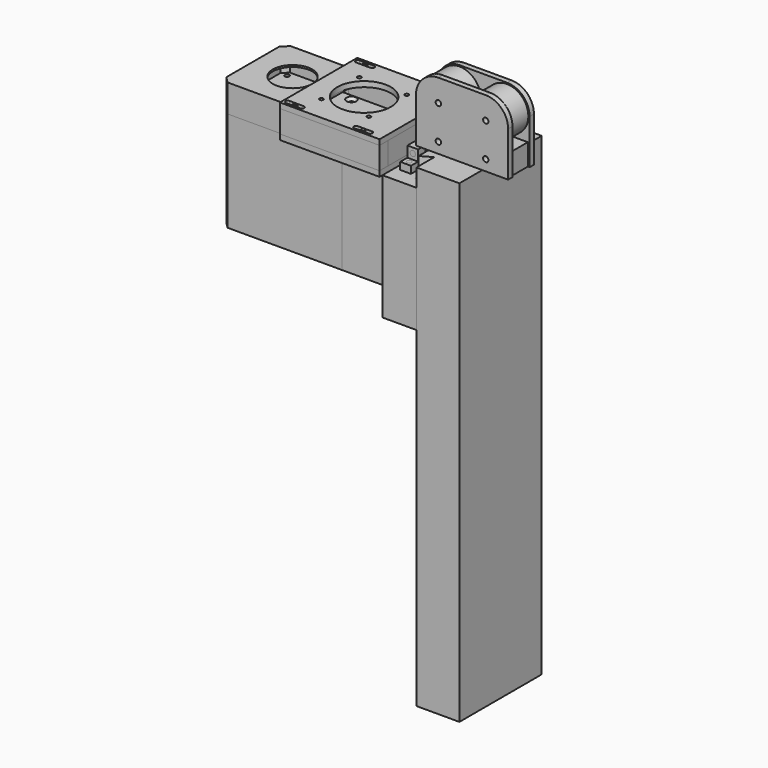
from build123d import *

# Parameters (mm, degrees)
F4_DEPTH       = 140
F1_W           = 50
F1_H           = 88
F1_R           = 2.5
F1_W_2         = 12
F1_H_2         = 10
F5_DEPTH       = 112
F1_R_2         = 25
F1_R_3         = 20
F6_DEPTH       = 112
F7_DEPTH       = 9.5
F8_DEPTH       = 9.5
F9_DEPTH       = 20
F2_R           = 2.5
F2_R_2         = 2.1
F2_R_3         = 6
F10_DEPTH      = 6
F11_SIZE       = 3
F3_W           = 101.8
F3_H           = 2
F3_W_2         = 9.6
F3_H_2         = 10
F3_R           = 2.1
F12_DEPTH      = 25
F3_H_3         = 84
F3_R_2         = 30
F13_DEPTH      = 6
F14_DEPTH      = 6
F14_DEPTH_BACK = 25
F15_DEPTH      = 25
F16_DEPTH      = 29
F17_R          = 25
F17_R_2        = 22
F18_DEPTH      = 2
F19_DEPTH      = 6
F21_DEPTH      = 1
F22_DEPTH      = 8
F23_DEPTH      = 20
F24_R          = 3
F25_DEPTH      = 45
F26_DEPTH      = 10
F27_DEPTH      = 8
F28_DEPTH      = 45
F30_DEPTH      = 20
F30_DEPTH_BACK = 510
F31_DEPTH      = 140
F29_W          = 5
F29_H          = 12.5
F29_W_2        = 2
F29_H_2        = 7.5
F32_DEPTH      = 380
F34_DEPTH      = 50
F35_R          = 24
F35_W          = 99
F35_H          = 24
F35_R_2        = 3
F35_R_3        = 11
F35_R_4        = 10
F35_R_5        = 4
F35_W_2        = 2
F36_DEPTH      = 18
F37_DEPTH      = 12
F38_DEPTH      = 12
F39_DEPTH      = 11.5
F40_DEPTH      = 5.5


with BuildPart() as f4:
    # F1 (on Top) → F4 (new body)
    with BuildSketch(Plane.XY):
        Polygon((0, -20), (0, 0), (-38, 0), (-38, -6), (-38, -94), (-38, -100), (0, -100), (0, -80), (-12.124355653, -87), (-12.124355653, -60), (-20.124355653, -60), (-20.124355653, -62.5), (-20.124355653, -72.5), (-20.124355653, -82.5), (-32.124355653, -82.5), (-32.124355653, -72.5), (-32.124355653, -62.5), (-32.124355653, -37.5), (-32.124355653, -27.5), (-32.124355653, -17.5), (-20.124355653, -17.5), (-20.124355653, -27.5), (-20.124355653, -35), (-12.124355653, -35), (-12.124355653, -13), align=None)
    extrude(amount=-F4_DEPTH)

    # F1 (on Top) → F5 (join)
    with BuildSketch(Plane.XY):
        with Locations((-63, -50)):
            Rectangle(F1_W, F1_H)
        with Locations((-55.6, -86)):
            Circle(F1_R, mode=Mode.SUBTRACT)
        with Locations((-55.6, -14)):
            Circle(F1_R, mode=Mode.SUBTRACT)
        Polygon((-20.124355653, -60), (-20.124355653, -37.5), (-32.124355653, -37.5), (-32.124355653, -62.5), (-20.124355653, -62.5), align=None)
        with Locations((-26.124355653, -50)):
            Circle(F1_R, mode=Mode.SUBTRACT)
        with Locations((-26.124355653, -77.5)):
            Rectangle(F1_W_2, F1_H_2)
        with Locations((-26.124355653, -77.5)):
            Circle(F1_R, mode=Mode.SUBTRACT)
        with Locations((-26.124355653, -22.5)):
            Rectangle(F1_W_2, F1_H_2)
        with Locations((-26.124355653, -22.5)):
            Circle(F1_R, mode=Mode.SUBTRACT)
        with Locations((-26.124355653, -67.5)):
            Rectangle(F1_W_2, F1_H_2)
        Polygon((-20.124355653, -37.5), (-20.124355653, -35), (-20.124355653, -27.5), (-32.124355653, -27.5), (-32.124355653, -37.5), align=None)
        with Locations((-55.6, -86)):
            Circle(F1_R)
        with Locations((-55.6, -14)):
            Circle(F1_R)
        with Locations((-26.124355653, -77.5)):
            Circle(F1_R)
        with Locations((-26.124355653, -50)):
            Circle(F1_R)
        with Locations((-26.124355653, -22.5)):
            Circle(F1_R)
    extrude(amount=-F5_DEPTH)


with BuildPart() as f6:
    # F1 (on Top) → F6 (new body)
    with BuildSketch(Plane.XY):
        Polygon((-88, -94), (-88, -6), (-215.9289321881, -6), (-223, -13.0710678119), (-223, -86.9289321881), (-215.9289321881, -94), align=None)
        with Locations((-213.4, -86)):
            Circle(F1_R, mode=Mode.SUBTRACT)
        with Locations((-141.4, -86)):
            Circle(F1_R, mode=Mode.SUBTRACT)
        with BuildLine():
            ThreePointArc((-140.061745502, -35.7346366626), (-126.6088552227, -37.8642844766), (-120.425, -50))
            ThreePointArc((-120.425, -50), (-126.6088552227, -62.1357155234), (-140.061745502, -64.2653633374))
            ThreePointArc((-140.061745502, -64.2653633374), (-219.5, -50), (-140.061745502, -35.7346366626))
        make_face(mode=Mode.SUBTRACT)
        with Locations((-213.4, -14)):
            Circle(F1_R, mode=Mode.SUBTRACT)
        with Locations((-141.4, -14)):
            Circle(F1_R, mode=Mode.SUBTRACT)
        with BuildLine():
            ThreePointArc((-140.061745502, -64.2653633374), (-150.425, -50), (-140.061745502, -35.7346366626))
            ThreePointArc((-140.061745502, -35.7346366626), (-219.5, -50), (-140.061745502, -64.2653633374))
        make_face()
        with Locations((-178.5, -50)):
            Circle(F1_R_2, mode=Mode.SUBTRACT)
        with BuildLine():
            ThreePointArc((-137.5, -50), (-138.1455180035, -42.7532225927), (-140.061745502, -35.7346366626))
            ThreePointArc((-140.061745502, -35.7346366626), (-150.425, -50), (-140.061745502, -64.2653633374))
            ThreePointArc((-140.061745502, -64.2653633374), (-138.1455180035, -57.2467774073), (-137.5, -50))
        make_face()
        with Locations((-178.5, -50)):
            Circle(F1_R_2)
        with Locations((-178.5, -50)):
            Circle(F1_R_3, mode=Mode.SUBTRACT)
        with BuildLine():
            ThreePointArc((-140.061745502, -64.2653633374), (-126.6088552227, -62.1357155234), (-120.425, -50))
            ThreePointArc((-120.425, -50), (-126.6088552227, -37.8642844766), (-140.061745502, -35.7346366626))
            ThreePointArc((-140.061745502, -35.7346366626), (-138.1455180035, -42.7532225927), (-137.5, -50))
            ThreePointArc((-137.5, -50), (-138.1455180035, -57.2467774073), (-140.061745502, -64.2653633374))
        make_face()
        with Locations((-141.4, -86)):
            Circle(F1_R)
        with Locations((-141.4, -14)):
            Circle(F1_R)
        with Locations((-213.4, -14)):
            Circle(F1_R)
        with Locations((-213.4, -86)):
            Circle(F1_R)
    extrude(amount=-F6_DEPTH)

    # F1 (on Top) → F7 (cut)
    with BuildSketch(Plane.XY):
        with BuildLine():
            ThreePointArc((-140.061745502, -64.2653633374), (-150.425, -50), (-140.061745502, -35.7346366626))
            ThreePointArc((-140.061745502, -35.7346366626), (-219.5, -50), (-140.061745502, -64.2653633374))
        make_face()
        with Locations((-178.5, -50)):
            Circle(F1_R_2, mode=Mode.SUBTRACT)
        with BuildLine():
            ThreePointArc((-137.5, -50), (-138.1455180035, -42.7532225927), (-140.061745502, -35.7346366626))
            ThreePointArc((-140.061745502, -35.7346366626), (-150.425, -50), (-140.061745502, -64.2653633374))
            ThreePointArc((-140.061745502, -64.2653633374), (-138.1455180035, -57.2467774073), (-137.5, -50))
        make_face()
        with BuildLine():
            ThreePointArc((-140.061745502, -64.2653633374), (-126.6088552227, -62.1357155234), (-120.425, -50))
            ThreePointArc((-120.425, -50), (-126.6088552227, -37.8642844766), (-140.061745502, -35.7346366626))
            ThreePointArc((-140.061745502, -35.7346366626), (-138.1455180035, -42.7532225927), (-137.5, -50))
            ThreePointArc((-137.5, -50), (-138.1455180035, -57.2467774073), (-140.061745502, -64.2653633374))
        make_face()
        with Locations((-178.5, -50)):
            Circle(F1_R_2)
        with Locations((-178.5, -50)):
            Circle(F1_R_3, mode=Mode.SUBTRACT)
    extrude(amount=-F7_DEPTH, mode=Mode.SUBTRACT)


with BuildPart() as f8:
    # F1 (on Top) → F8 (new body, through all)
    with BuildSketch(Plane.XY):
        with BuildLine():
            ThreePointArc((-140.061745502, -64.2653633374), (-150.425, -50), (-140.061745502, -35.7346366626))
            ThreePointArc((-140.061745502, -35.7346366626), (-219.5, -50), (-140.061745502, -64.2653633374))
        make_face()
        with Locations((-178.5, -50)):
            Circle(F1_R_2, mode=Mode.SUBTRACT)
    extrude(amount=-F8_DEPTH)


with BuildPart() as f9_tool:
    # F1 (on Top) → F9 (new body)
    with BuildSketch(Plane.XY):
        with Locations((-213.4, -14)):
            Circle(F1_R)
        with Locations((-55.6, -14)):
            Circle(F1_R)
        with Locations((-55.6, -86)):
            Circle(F1_R)
        with Locations((-213.4, -86)):
            Circle(F1_R)
        with Locations((-141.4, -86)):
            Circle(F1_R)
        with Locations((-141.4, -14)):
            Circle(F1_R)
    extrude(amount=-F9_DEPTH)


with BuildPart() as f4_1:
    add(f4.part)

    # F9: cut by f9_tool
    add(f9_tool.part, mode=Mode.SUBTRACT)

    # F1 (on Top) → F26 (cut)
    with BuildSketch(Plane.XY):
        with Locations((-26.124355653, -77.5)):
            Circle(F1_R)
        with Locations((-26.124355653, -50)):
            Circle(F1_R)
        with Locations((-26.124355653, -22.5)):
            Circle(F1_R)
    extrude(amount=-F26_DEPTH, mode=Mode.SUBTRACT)


with BuildPart() as f6_1:
    add(f6.part)

    # F9: cut by f9_tool
    add(f9_tool.part, mode=Mode.SUBTRACT)


with BuildPart() as f10:
    # F2 (on Top) → F10 (new body)
    with BuildSketch(Plane.XY):
        with BuildLine():
            Line((-175.5, -25), (-175.5, -8))
            Line((-175.5, -8), (-181.5, -8))
            Line((-181.5, -8), (-181.5, -25.180652708))
            ThreePointArc((-181.5, -25.180652708), (-180.0027171558, -25.0452040451), (-178.5, -25))
            Line((-178.5, -25), (-175.5, -25))
        make_face()
        with BuildLine():
            Line((-47.6, -6), (-88, -6))
            Line((-88, -6), (-149.4, -6))
            Line((-149.4, -6), (-149.4, -8))
            Line((-149.4, -8), (-175.5, -8))
            Line((-175.5, -8), (-175.5, -25))
            Line((-175.5, -25), (-98.5, -25))
            ThreePointArc((-98.5, -25), (-80.8223304703, -32.3223304703), (-73.5, -50))
            ThreePointArc((-73.5, -50), (-80.8223304703, -67.6776695297), (-98.5, -75))
            Line((-98.5, -75), (-178.5, -75))
            ThreePointArc((-178.5, -75), (-203.4547959549, -51.5027171558), (-181.5, -25.180652708))
            Line((-181.5, -25.180652708), (-181.5, -8))
            Line((-181.5, -8), (-215.1005050634, -8))
            Line((-215.1005050634, -8), (-221, -13.8994949366))
            Line((-221, -13.8994949366), (-221, -86.1005050634))
            Line((-221, -86.1005050634), (-215.1005050634, -92))
            Line((-215.1005050634, -92), (-149.4, -92))
            Line((-149.4, -92), (-149.4, -94))
            Line((-149.4, -94), (-88, -94))
            Line((-88, -94), (-47.6, -94))
            Line((-47.6, -94), (-47.6, -6))
        make_face()
        with Locations((-213.4, -86)):
            Circle(F2_R, mode=Mode.SUBTRACT)
        with Locations((-141.4, -86)):
            Circle(F2_R, mode=Mode.SUBTRACT)
        with Locations((-55.6, -86)):
            Circle(F2_R, mode=Mode.SUBTRACT)
        with Locations((-213.4, -14)):
            Circle(F2_R, mode=Mode.SUBTRACT)
        with Locations((-141.4, -14)):
            Circle(F2_R, mode=Mode.SUBTRACT)
        with Locations((-55.6, -14)):
            Circle(F2_R, mode=Mode.SUBTRACT)
        Polygon((-149.4, -6), (-88, -6), (-47.6, -6), (-47.6, 4), (-88, 4), (-149.4, 4), align=None)
        with Locations((-144.687037037, -1)):
            Circle(F2_R, mode=Mode.SUBTRACT)
        with Locations((-136.687037037, -1)):
            Circle(F2_R_2, mode=Mode.SUBTRACT)
        with Locations((-128.687037037, -1)):
            Circle(F2_R, mode=Mode.SUBTRACT)
        with Locations((-60.312962963, -1)):
            Circle(F2_R_2, mode=Mode.SUBTRACT)
        with Locations((-52.312962963, -1)):
            Circle(F2_R, mode=Mode.SUBTRACT)
        Polygon((-47.6, -104), (-47.6, -94), (-88, -94), (-149.4, -94), (-149.4, -104), (-88, -104), align=None)
        with Locations((-144.687037037, -99)):
            Circle(F2_R, mode=Mode.SUBTRACT)
        with Locations((-136.687037037, -99)):
            Circle(F2_R_2, mode=Mode.SUBTRACT)
        with Locations((-128.687037037, -99)):
            Circle(F2_R, mode=Mode.SUBTRACT)
        with Locations((-60.312962963, -99)):
            Circle(F2_R_2, mode=Mode.SUBTRACT)
        with Locations((-52.312962963, -99)):
            Circle(F2_R, mode=Mode.SUBTRACT)
        with Locations((-60.312962963, -1)):
            Circle(F2_R_2)
        with Locations((-60.312962963, -99)):
            Circle(F2_R_2)
        with Locations((-136.687037037, -1)):
            Circle(F2_R_2)
        with Locations((-136.687037037, -99)):
            Circle(F2_R_2)
        Polygon((-47.6, 4), (-47.6, -6), (-47.6, -94), (-47.6, -104), (-38, -104), (-38, -94), (-38, -6), (-38, 4), align=None)
        with BuildLine():
            ThreePointArc((-73.5, -50), (-80.8223304703, -32.3223304703), (-98.5, -25))
            ThreePointArc((-98.5, -25), (-113.3312903934, -29.8745726687), (-122.3788845633, -42.5973739786))
            ThreePointArc((-122.3788845633, -42.5973739786), (-120.9216946603, -46.1719281322), (-120.425, -50))
            ThreePointArc((-120.425, -50), (-120.9216946603, -53.8280718678), (-122.3788845633, -57.4026260214))
            ThreePointArc((-122.3788845633, -57.4026260214), (-113.3312903934, -70.1254273313), (-98.5, -75))
            ThreePointArc((-98.5, -75), (-80.8223304703, -67.6776695297), (-73.5, -50))
        make_face()
        with BuildLine():
            Line((-98.5, -25), (-175.5, -25))
            Line((-175.5, -25), (-175.5, -25.180652708))
            ThreePointArc((-175.5, -25.180652708), (-159.7917130661, -33.4168760482), (-153.5, -50))
            ThreePointArc((-153.5, -50), (-160.8223304703, -67.6776695297), (-178.5, -75))
            Line((-178.5, -75), (-98.5, -75))
            ThreePointArc((-98.5, -75), (-113.3312903934, -70.1254273313), (-122.3788845633, -57.4026260214))
            ThreePointArc((-122.3788845633, -57.4026260214), (-150.425, -50), (-122.3788845633, -42.5973739786))
            ThreePointArc((-122.3788845633, -42.5973739786), (-113.3312903934, -29.8745726687), (-98.5, -25))
        make_face()
        with BuildLine():
            ThreePointArc((-122.3788845633, -57.4026260214), (-123.5, -50), (-122.3788845633, -42.5973739786))
            ThreePointArc((-122.3788845633, -42.5973739786), (-150.425, -50), (-122.3788845633, -57.4026260214))
        make_face()
        with Locations((-135.425, -50)):
            Circle(F2_R_3, mode=Mode.SUBTRACT)
        with BuildLine():
            ThreePointArc((-120.425, -50), (-120.9216946603, -46.1719281322), (-122.3788845633, -42.5973739786))
            ThreePointArc((-122.3788845633, -42.5973739786), (-123.5, -50), (-122.3788845633, -57.4026260214))
            ThreePointArc((-122.3788845633, -57.4026260214), (-120.9216946603, -53.8280718678), (-120.425, -50))
        make_face()
    extrude(amount=F10_DEPTH)

    # F11
    f11_edges = [f10.edges().sort_by_distance(p)[0] for p in [
        (-143.9, -14, 6),
        (-143.9, -86, 6),
    ]]
    chamfer(f11_edges, length=F11_SIZE)

    # F2 (on Top) → F19 (cut, through all)
    with BuildSketch(Plane.XY):
        with BuildLine():
            Line((-175.5, -25), (-175.5, -8))
            Line((-175.5, -8), (-181.5, -8))
            Line((-181.5, -8), (-181.5, -25.180652708))
            ThreePointArc((-181.5, -25.180652708), (-180.0027171558, -25.0452040451), (-178.5, -25))
            Line((-178.5, -25), (-175.5, -25))
        make_face()
    extrude(amount=F19_DEPTH, mode=Mode.SUBTRACT)

    # F20 (on face) → F21 (join)
    with BuildSketch(Plane.XY.offset(6)):
        with BuildLine():
            Line((-181.5, -8), (-183.5, -8))
            Line((-183.5, -8), (-183.5, -25.5051025722))
            ThreePointArc((-183.5, -25.5051025722), (-182.5032882645, -25.3226078551), (-181.5, -25.180652708))
            Line((-181.5, -25.180652708), (-181.5, -8))
        make_face()
        with BuildLine():
            Line((-173.5, -8), (-175.5, -8))
            Line((-175.5, -8), (-175.5, -25.180652708))
            ThreePointArc((-175.5, -25.180652708), (-174.4967117355, -25.3226078551), (-173.5, -25.5051025722))
            Line((-173.5, -25.5051025722), (-173.5, -8))
        make_face()
        with BuildLine():
            Line((-175.5, -8), (-181.5, -8))
            Line((-181.5, -8), (-181.5, -25.180652708))
            ThreePointArc((-181.5, -25.180652708), (-178.5, -25), (-175.5, -25.180652708))
            Line((-175.5, -25.180652708), (-175.5, -8))
        make_face()
    extrude(amount=F21_DEPTH)


with BuildPart() as f12:
    # F3 (on offset) → F12 (new body)
    with BuildSketch(Plane.XY.offset(31)):
        Polygon((-47.6, -94), (-149.4, -94), (-149.4, -104), (-88, -104), (-47.6, -104), align=None)
        with BuildLine():
            ThreePointArc((-144.687037037, -101.5), (-147.187037037, -99), (-144.687037037, -96.5))
            Line((-144.687037037, -96.5), (-128.687037037, -96.5))
            ThreePointArc((-128.687037037, -96.5), (-126.9192700841, -97.232233047), (-126.187037037, -99))
            ThreePointArc((-126.187037037, -99), (-126.9192700841, -100.767766953), (-128.687037037, -101.5))
            Line((-128.687037037, -101.5), (-144.687037037, -101.5))
        make_face(mode=Mode.SUBTRACT)
        with BuildLine():
            ThreePointArc((-52.312962963, -96.5), (-50.54519601, -97.232233047), (-49.812962963, -99))
            ThreePointArc((-49.812962963, -99), (-50.54519601, -100.767766953), (-52.312962963, -101.5))
            Line((-52.312962963, -101.5), (-68.312962963, -101.5))
            ThreePointArc((-68.312962963, -101.5), (-70.812962963, -99), (-68.312962963, -96.5))
            Line((-68.312962963, -96.5), (-52.312962963, -96.5))
        make_face(mode=Mode.SUBTRACT)
        with Locations((-98.5, -93)):
            Rectangle(F3_W, F3_H)
        with Locations((-42.8, -99)):
            Rectangle(F3_W_2, F3_H_2)
        with BuildLine():
            ThreePointArc((-52.312962963, -101.5), (-54.812962963, -99), (-52.312962963, -96.5))
            Line((-52.312962963, -96.5), (-68.312962963, -96.5))
            ThreePointArc((-68.312962963, -96.5), (-66.54519601, -97.232233047), (-65.812962963, -99))
            ThreePointArc((-65.812962963, -99), (-66.54519601, -100.767766953), (-68.312962963, -101.5))
            Line((-68.312962963, -101.5), (-52.312962963, -101.5))
        make_face()
        with Locations((-60.312962963, -99)):
            Circle(F3_R, mode=Mode.SUBTRACT)
        with BuildLine():
            ThreePointArc((-144.687037037, -96.5), (-142.9192700841, -97.232233047), (-142.187037037, -99))
            ThreePointArc((-142.187037037, -99), (-142.9192700841, -100.767766953), (-144.687037037, -101.5))
            Line((-144.687037037, -101.5), (-128.687037037, -101.5))
            ThreePointArc((-128.687037037, -101.5), (-131.187037037, -99), (-128.687037037, -96.5))
            Line((-128.687037037, -96.5), (-144.687037037, -96.5))
        make_face()
        with Locations((-136.687037037, -99)):
            Circle(F3_R, mode=Mode.SUBTRACT)
        with BuildLine():
            ThreePointArc((-65.812962963, -99), (-66.54519601, -97.232233047), (-68.312962963, -96.5))
            ThreePointArc((-68.312962963, -96.5), (-70.812962963, -99), (-68.312962963, -101.5))
            ThreePointArc((-68.312962963, -101.5), (-66.54519601, -100.767766953), (-65.812962963, -99))
        make_face()
        with Locations((-42.8, -93)):
            Rectangle(F3_W_2, F3_H)
    extrude(amount=-F12_DEPTH)


with BuildPart() as f12b:
    # F3 (on offset) → F12, piece 2 (new body)
    with BuildSketch(Plane.XY.offset(31)):
        Polygon((-47.6, 4), (-88, 4), (-149.4, 4), (-149.4, -6), (-47.6, -6), align=None)
        with BuildLine():
            ThreePointArc((-144.687037037, -3.5), (-147.187037037, -1), (-144.687037037, 1.5))
            Line((-144.687037037, 1.5), (-128.687037037, 1.5))
            ThreePointArc((-128.687037037, 1.5), (-126.9192700841, 0.767766953), (-126.187037037, -1))
            ThreePointArc((-126.187037037, -1), (-126.9192700841, -2.767766953), (-128.687037037, -3.5))
            Line((-128.687037037, -3.5), (-144.687037037, -3.5))
        make_face(mode=Mode.SUBTRACT)
        with BuildLine():
            ThreePointArc((-52.312962963, 1.5), (-50.54519601, 0.767766953), (-49.812962963, -1))
            ThreePointArc((-49.812962963, -1), (-50.54519601, -2.767766953), (-52.312962963, -3.5))
            Line((-52.312962963, -3.5), (-68.312962963, -3.5))
            ThreePointArc((-68.312962963, -3.5), (-70.812962963, -1), (-68.312962963, 1.5))
            Line((-68.312962963, 1.5), (-52.312962963, 1.5))
        make_face(mode=Mode.SUBTRACT)
        with Locations((-98.5, -7)):
            Rectangle(F3_W, F3_H)
        with Locations((-42.8, -1)):
            Rectangle(F3_W_2, F3_H_2)
        with BuildLine():
            ThreePointArc((-52.312962963, -3.5), (-54.812962963, -1), (-52.312962963, 1.5))
            Line((-52.312962963, 1.5), (-68.312962963, 1.5))
            ThreePointArc((-68.312962963, 1.5), (-66.54519601, 0.767766953), (-65.812962963, -1))
            ThreePointArc((-65.812962963, -1), (-66.54519601, -2.767766953), (-68.312962963, -3.5))
            Line((-68.312962963, -3.5), (-52.312962963, -3.5))
        make_face()
        with Locations((-60.312962963, -1)):
            Circle(F3_R, mode=Mode.SUBTRACT)
        with BuildLine():
            ThreePointArc((-144.687037037, 1.5), (-142.9192700841, 0.767766953), (-142.187037037, -1))
            ThreePointArc((-142.187037037, -1), (-142.9192700841, -2.767766953), (-144.687037037, -3.5))
            Line((-144.687037037, -3.5), (-128.687037037, -3.5))
            ThreePointArc((-128.687037037, -3.5), (-131.187037037, -1), (-128.687037037, 1.5))
            Line((-128.687037037, 1.5), (-144.687037037, 1.5))
        make_face()
        with Locations((-136.687037037, -1)):
            Circle(F3_R, mode=Mode.SUBTRACT)
        with BuildLine():
            ThreePointArc((-65.812962963, -1), (-66.54519601, 0.767766953), (-68.312962963, 1.5))
            ThreePointArc((-68.312962963, 1.5), (-70.812962963, -1), (-68.312962963, -3.5))
            ThreePointArc((-68.312962963, -3.5), (-66.54519601, -2.767766953), (-65.812962963, -1))
        make_face()
        with Locations((-42.8, -7)):
            Rectangle(F3_W_2, F3_H)
    extrude(amount=-F12_DEPTH)


with BuildPart() as f13:
    # F3 (on offset) → F13 (new body)
    with BuildSketch(Plane.XY.offset(31)):
        Polygon((-47.6, 4), (-88, 4), (-149.4, 4), (-149.4, -6), (-47.6, -6), align=None)
        with BuildLine():
            ThreePointArc((-144.687037037, -3.5), (-147.187037037, -1), (-144.687037037, 1.5))
            Line((-144.687037037, 1.5), (-128.687037037, 1.5))
            ThreePointArc((-128.687037037, 1.5), (-126.9192700841, 0.767766953), (-126.187037037, -1))
            ThreePointArc((-126.187037037, -1), (-126.9192700841, -2.767766953), (-128.687037037, -3.5))
            Line((-128.687037037, -3.5), (-144.687037037, -3.5))
        make_face(mode=Mode.SUBTRACT)
        with BuildLine():
            ThreePointArc((-52.312962963, 1.5), (-50.54519601, 0.767766953), (-49.812962963, -1))
            ThreePointArc((-49.812962963, -1), (-50.54519601, -2.767766953), (-52.312962963, -3.5))
            Line((-52.312962963, -3.5), (-68.312962963, -3.5))
            ThreePointArc((-68.312962963, -3.5), (-70.812962963, -1), (-68.312962963, 1.5))
            Line((-68.312962963, 1.5), (-52.312962963, 1.5))
        make_face(mode=Mode.SUBTRACT)
        with Locations((-98.5, -7)):
            Rectangle(F3_W, F3_H)
        with Locations((-98.5, -50)):
            Rectangle(F3_W, F3_H_3)
        with Locations((-125.0165042945, -76.5165042945)):
            Circle(F3_R, mode=Mode.SUBTRACT)
        with Locations((-71.9834957055, -76.5165042945)):
            Circle(F3_R, mode=Mode.SUBTRACT)
        with Locations((-125.0165042945, -23.4834957055)):
            Circle(F3_R, mode=Mode.SUBTRACT)
        with Locations((-98.5, -50)):
            Circle(F3_R_2, mode=Mode.SUBTRACT)
        with Locations((-71.9834957055, -23.4834957055)):
            Circle(F3_R, mode=Mode.SUBTRACT)
        with Locations((-98.5, -93)):
            Rectangle(F3_W, F3_H)
        Polygon((-47.6, -94), (-149.4, -94), (-149.4, -104), (-88, -104), (-47.6, -104), align=None)
        with BuildLine():
            ThreePointArc((-144.687037037, -101.5), (-147.187037037, -99), (-144.687037037, -96.5))
            Line((-144.687037037, -96.5), (-128.687037037, -96.5))
            ThreePointArc((-128.687037037, -96.5), (-126.9192700841, -97.232233047), (-126.187037037, -99))
            ThreePointArc((-126.187037037, -99), (-126.9192700841, -100.767766953), (-128.687037037, -101.5))
            Line((-128.687037037, -101.5), (-144.687037037, -101.5))
        make_face(mode=Mode.SUBTRACT)
        with BuildLine():
            ThreePointArc((-52.312962963, -96.5), (-50.54519601, -97.232233047), (-49.812962963, -99))
            ThreePointArc((-49.812962963, -99), (-50.54519601, -100.767766953), (-52.312962963, -101.5))
            Line((-52.312962963, -101.5), (-68.312962963, -101.5))
            ThreePointArc((-68.312962963, -101.5), (-70.812962963, -99), (-68.312962963, -96.5))
            Line((-68.312962963, -96.5), (-52.312962963, -96.5))
        make_face(mode=Mode.SUBTRACT)
        with Locations((-42.8, -7)):
            Rectangle(F3_W_2, F3_H)
        with Locations((-42.8, -50)):
            Rectangle(F3_W_2, F3_H_3)
        with Locations((-42.8, -93)):
            Rectangle(F3_W_2, F3_H)
        with Locations((-42.8, -99)):
            Rectangle(F3_W_2, F3_H_2)
        with Locations((-42.8, -1)):
            Rectangle(F3_W_2, F3_H_2)
    extrude(amount=F13_DEPTH)


with BuildPart() as f14:
    # F3 (on offset) → F14 (new body, two sides)
    with BuildSketch(Plane.XY.offset(31)) as f14_sk:
        with Locations((-136.687037037, -99)):
            Circle(F3_R)
    extrude(amount=F14_DEPTH)
    extrude(f14_sk.sketch, amount=-F14_DEPTH_BACK)


with BuildPart() as f14b:
    # F3 (on offset) → F14, piece 2 (new body, two sides)
    with BuildSketch(Plane.XY.offset(31)) as f14_2_sk:
        with Locations((-136.687037037, -1)):
            Circle(F3_R)
    extrude(amount=F14_DEPTH)
    extrude(f14_2_sk.sketch, amount=-F14_DEPTH_BACK)


with BuildPart() as f14c:
    # F3 (on offset) → F14, piece 3 (new body, two sides)
    with BuildSketch(Plane.XY.offset(31)) as f14_3_sk:
        with Locations((-60.312962963, -1)):
            Circle(F3_R)
    extrude(amount=F14_DEPTH)
    extrude(f14_3_sk.sketch, amount=-F14_DEPTH_BACK)


with BuildPart() as f14d:
    # F3 (on offset) → F14, piece 4 (new body, two sides)
    with BuildSketch(Plane.XY.offset(31)) as f14_4_sk:
        with Locations((-60.312962963, -99)):
            Circle(F3_R)
    extrude(amount=F14_DEPTH)
    extrude(f14_4_sk.sketch, amount=-F14_DEPTH_BACK)


with BuildPart() as f15:
    # F3 (on offset) → F15 (new body)
    with BuildSketch(Plane.XY.offset(31)):
        with Locations((-42.8, -50)):
            Rectangle(F3_W_2, F3_H_3)
    extrude(amount=-F15_DEPTH)


with BuildPart() as f16:
    # F2 (on Top) → F16 (new body)
    with BuildSketch(Plane.XY):
        Polygon((-149.4, -8), (-149.4, -6), (-215.9289321881, -6), (-223, -13.0710678119), (-223, -86.9289321881), (-215.9289321881, -94), (-149.4, -94), (-149.4, -92), (-215.1005050634, -92), (-221, -86.1005050634), (-221, -13.8994949366), (-215.1005050634, -8), (-181.5, -8), (-175.5, -8), align=None)
    extrude(amount=F16_DEPTH)

    # F17 (on face) → F18 (join)
    with BuildSketch(Plane.XY.offset(29)):
        Polygon((-149.4, -92), (-149.4, -8), (-215.1005050634, -8), (-221, -13.8994949366), (-221, -86.1005050634), (-215.1005050634, -92), align=None)
        with Locations((-178.5, -50)):
            Circle(F17_R, mode=Mode.SUBTRACT)
        with Locations((-178.5, -50)):
            Circle(F17_R)
        with Locations((-178.5, -50)):
            Circle(F17_R_2, mode=Mode.SUBTRACT)
        with BuildLine():
            ThreePointArc((-128.5, -16.4589803375), (-139.5791918129, -31.6288269291), (-143.5, -50))
            ThreePointArc((-143.5, -50), (-139.5791918129, -68.3711730709), (-128.5, -83.5410196625))
            Line((-128.5, -83.5410196625), (-128.5, -50))
            Line((-128.5, -50), (-128.5, -16.4589803375))
        make_face()
        Polygon((-143.5, -8), (-149.4, -8), (-149.4, -92), (-143.5, -92), (-143.5, -50), align=None)
        Polygon((-149.4, -6), (-215.9289321881, -6), (-223, -13.0710678119), (-223, -86.9289321881), (-215.9289321881, -94), (-149.4, -94), (-149.4, -92), (-215.1005050634, -92), (-221, -86.1005050634), (-221, -13.8994949366), (-215.1005050634, -8), (-149.4, -8), align=None)
        with BuildLine():
            Line((-128.5, -8), (-143.5, -8))
            Line((-143.5, -8), (-143.5, -50))
            ThreePointArc((-143.5, -50), (-139.5791918129, -31.6288269291), (-128.5, -16.4589803375))
            Line((-128.5, -16.4589803375), (-128.5, -8))
        make_face()
        with BuildLine():
            ThreePointArc((-128.5, -83.5410196625), (-139.5791918129, -68.3711730709), (-143.5, -50))
            Line((-143.5, -50), (-143.5, -92))
            Line((-143.5, -92), (-128.5, -92))
            Line((-128.5, -92), (-128.5, -83.5410196625))
        make_face()
    extrude(amount=F18_DEPTH)


with BuildPart() as f22:
    # F1 (on Top) → F22 (new body)
    with BuildSketch(Plane.XY):
        with Locations((-26.124355653, -22.5)):
            Rectangle(F1_W_2, F1_H_2)
        with Locations((-26.124355653, -22.5)):
            Circle(F1_R, mode=Mode.SUBTRACT)
    extrude(amount=F22_DEPTH)



with BuildPart() as f22b:
    # F1 (on Top) → F22, piece 2 (new body)
    with BuildSketch(Plane.XY):
        Polygon((-20.124355653, -60), (-20.124355653, -37.5), (-32.124355653, -37.5), (-32.124355653, -62.5), (-20.124355653, -62.5), align=None)
        with Locations((-26.124355653, -50)):
            Circle(F1_R, mode=Mode.SUBTRACT)
    extrude(amount=F22_DEPTH)


with BuildPart() as f22c:
    # F1 (on Top) → F22, piece 3 (new body)
    with BuildSketch(Plane.XY):
        with Locations((-26.124355653, -77.5)):
            Rectangle(F1_W_2, F1_H_2)
        with Locations((-26.124355653, -77.5)):
            Circle(F1_R, mode=Mode.SUBTRACT)
    extrude(amount=F22_DEPTH)


with BuildPart() as f22_1:
    add(f22.part)

    add(f22b.part)  # F23 merges F22b

    add(f22c.part)  # F23 merges F22c
    # F1 (on Top) → F23 (join)
    with BuildSketch(Plane.XY):
        Polygon((-20.124355653, -37.5), (-20.124355653, -35), (-20.124355653, -27.5), (-32.124355653, -27.5), (-32.124355653, -37.5), align=None)
        with Locations((-26.124355653, -67.5)):
            Rectangle(F1_W_2, F1_H_2)
    extrude(amount=F23_DEPTH)

    # F24 (on face) → F25 (cut, through all)
    with BuildSketch(Plane.XZ.offset(72.5)):
        with Locations((-26.124355653, 14)):
            Circle(F24_R)
    extrude(amount=-F25_DEPTH, mode=Mode.SUBTRACT)


with BuildPart() as f27:
    # F1 (on Top) → F27 (new body, symmetric)
    with BuildSketch(Plane.XY):
        with Locations((-26.124355653, -77.5)):
            Circle(F1_R)
    extrude(amount=F27_DEPTH, both=True)


with BuildPart() as f27b:
    # F1 (on Top) → F27, piece 2 (new body, symmetric)
    with BuildSketch(Plane.XY):
        with Locations((-26.124355653, -50)):
            Circle(F1_R)
    extrude(amount=F27_DEPTH, both=True)


with BuildPart() as f27c:
    # F1 (on Top) → F27, piece 3 (new body, symmetric)
    with BuildSketch(Plane.XY):
        with Locations((-26.124355653, -22.5)):
            Circle(F1_R)
    extrude(amount=F27_DEPTH, both=True)


with BuildPart() as f28:
    # F24 (on face) → F28 (new body, through all)
    with BuildSketch(Plane.XZ.offset(72.5)):
        with Locations((-26.124355653, 14)):
            Circle(F24_R)
    extrude(amount=-F28_DEPTH)


with BuildPart() as f30:
    # F29 (on face) → F30 (new body, two sides)
    with BuildSketch(Plane.XY) as f30_sk:
        Polygon((0, -20), (-12.124355653, -13), (-12.124355653, -35), (-12.124355653, -37.5), (-7.124355653, -37.5), (-7.124355653, -50), (-7.124355653, -57.5), (-12.124355653, -57.5), (-12.124355653, -60), (-12.124355653, -82), (0, -75), (0, -80), (0, -100), (48, -100), (48, 15), (4, 15), (0, 4.753049234), (0, 0), align=None)
    extrude(amount=F30_DEPTH)
    extrude(f30_sk.sketch, amount=-F30_DEPTH_BACK)


with BuildPart() as f31:
    # F29 (on face) → F31 (new body, through all)
    with BuildSketch(Plane.XY):
        Polygon((0, -75), (-12.124355653, -82), (-12.124355653, -87), (0, -80), align=None)
    extrude(amount=-F31_DEPTH)


with BuildPart() as f32:
    # F29 (on face) → F32 (new body)
    with BuildSketch(Plane.XY):
        with Locations((-9.624355653, -43.75)):
            Rectangle(F29_W, F29_H)
        with Locations((-13.124355653, -43.75)):
            Rectangle(F29_W_2, F29_H)
        with Locations((-13.124355653, -53.75)):
            Rectangle(F29_W_2, F29_H_2)
        with Locations((-9.624355653, -53.75)):
            Rectangle(F29_W, F29_H_2)
    extrude(amount=-F32_DEPTH)

    # F29 (on face) → F34 (cut)
    with BuildSketch(Plane.XY):
        with Locations((-9.624355653, -43.75)):
            Rectangle(F29_W, F29_H)
        with Locations((-13.124355653, -43.75)):
            Rectangle(F29_W_2, F29_H)
        with Locations((-13.124355653, -53.75)):
            Rectangle(F29_W_2, F29_H_2)
        Polygon((-12.124355653, -37.5), (-12.124355653, -35), (-20.124355653, -35), (-20.124355653, -60), (-12.124355653, -60), (-12.124355653, -57.5), (-14.124355653, -57.5), (-14.124355653, -50), (-14.124355653, -37.5), align=None)
        with Locations((-9.624355653, -53.75)):
            Rectangle(F29_W, F29_H_2)
    extrude(amount=-F34_DEPTH, mode=Mode.SUBTRACT)


with BuildPart() as f36:
    # F35 (on line) → F36 (new body, symmetric)
    with BuildSketch(Plane.XZ.offset(50)):
        with BuildLine():
            Line((51.875644347, 95), (-1.124355653, 95))
            ThreePointArc((-1.124355653, 95), (-18.8020251826, 87.6776695297), (-26.124355653, 70))
            Line((-26.124355653, 70), (-26.124355653, 44))
            Line((-26.124355653, 44), (-24.124355653, 44))
            Line((-24.124355653, 44), (74.875644347, 44))
            Line((74.875644347, 44), (76.875644347, 44))
            Line((76.875644347, 44), (76.875644347, 70))
            ThreePointArc((76.875644347, 70), (69.5533138767, 87.6776695297), (51.875644347, 95))
        make_face()
        with Locations((-1.124355653, 70)):
            Circle(F35_R, mode=Mode.SUBTRACT)
        with Locations((51.875644347, 70)):
            Circle(F35_R, mode=Mode.SUBTRACT)
        with Locations((25.375644347, 32)):
            Rectangle(F35_W, F35_H)
        with Locations((-1.124355653, 32)):
            Circle(F35_R_2, mode=Mode.SUBTRACT)
        with Locations((51.875644347, 32)):
            Circle(F35_R_2, mode=Mode.SUBTRACT)
        with Locations((-1.124355653, 70)):
            Circle(F35_R)
        with Locations((-1.124355653, 70)):
            Circle(F35_R_3, mode=Mode.SUBTRACT)
        with Locations((51.875644347, 70)):
            Circle(F35_R)
        with Locations((51.875644347, 70)):
            Circle(F35_R_3, mode=Mode.SUBTRACT)
        with Locations((-1.124355653, 70)):
            Circle(F35_R_3)
        with Locations((-1.124355653, 70)):
            Circle(F35_R_4, mode=Mode.SUBTRACT)
        with Locations((51.875644347, 70)):
            Circle(F35_R_3)
        with Locations((51.875644347, 70)):
            Circle(F35_R_4, mode=Mode.SUBTRACT)
        with Locations((-1.124355653, 70)):
            Circle(F35_R_4)
        with Locations((-1.124355653, 70)):
            Circle(F35_R_5, mode=Mode.SUBTRACT)
        with Locations((51.875644347, 70)):
            Circle(F35_R_4)
        with Locations((51.875644347, 70)):
            Circle(F35_R_5, mode=Mode.SUBTRACT)
        with Locations((-1.124355653, 70)):
            Circle(F35_R_5)
        with Locations((-1.124355653, 70)):
            Circle(F35_R_2, mode=Mode.SUBTRACT)
        with Locations((51.875644347, 70)):
            Circle(F35_R_5)
        with Locations((51.875644347, 70)):
            Circle(F35_R_2, mode=Mode.SUBTRACT)
        with Locations((75.875644347, 32)):
            Rectangle(F35_W_2, F35_H)
        with Locations((-25.124355653, 32)):
            Rectangle(F35_W_2, F35_H)
    extrude(amount=F36_DEPTH, both=True)


with BuildPart() as f37:
    # F35 (on line) → F37 (new body, symmetric)
    with BuildSketch(Plane.XZ.offset(50)):
        with BuildLine():
            Line((51.875644347, 95), (-1.124355653, 95))
            ThreePointArc((-1.124355653, 95), (-18.8020251826, 87.6776695297), (-26.124355653, 70))
            Line((-26.124355653, 70), (-26.124355653, 44))
            Line((-26.124355653, 44), (-24.124355653, 44))
            Line((-24.124355653, 44), (74.875644347, 44))
            Line((74.875644347, 44), (76.875644347, 44))
            Line((76.875644347, 44), (76.875644347, 70))
            ThreePointArc((76.875644347, 70), (69.5533138767, 87.6776695297), (51.875644347, 95))
        make_face()
        with Locations((-1.124355653, 70)):
            Circle(F35_R, mode=Mode.SUBTRACT)
        with Locations((51.875644347, 70)):
            Circle(F35_R, mode=Mode.SUBTRACT)
        with Locations((25.375644347, 32)):
            Rectangle(F35_W, F35_H)
        with Locations((-1.124355653, 32)):
            Circle(F35_R_2, mode=Mode.SUBTRACT)
        with Locations((51.875644347, 32)):
            Circle(F35_R_2, mode=Mode.SUBTRACT)
        with Locations((51.875644347, 70)):
            Circle(F35_R)
        with Locations((51.875644347, 70)):
            Circle(F35_R_3, mode=Mode.SUBTRACT)
        with Locations((-1.124355653, 70)):
            Circle(F35_R)
        with Locations((-1.124355653, 70)):
            Circle(F35_R_3, mode=Mode.SUBTRACT)
        with Locations((51.875644347, 70)):
            Circle(F35_R_3)
        with Locations((51.875644347, 70)):
            Circle(F35_R_4, mode=Mode.SUBTRACT)
        with Locations((-1.124355653, 70)):
            Circle(F35_R_3)
        with Locations((-1.124355653, 70)):
            Circle(F35_R_4, mode=Mode.SUBTRACT)
        with Locations((-1.124355653, 70)):
            Circle(F35_R_4)
        with Locations((-1.124355653, 70)):
            Circle(F35_R_5, mode=Mode.SUBTRACT)
        with Locations((51.875644347, 70)):
            Circle(F35_R_4)
        with Locations((51.875644347, 70)):
            Circle(F35_R_5, mode=Mode.SUBTRACT)
        with Locations((-1.124355653, 70)):
            Circle(F35_R_5)
        with Locations((-1.124355653, 70)):
            Circle(F35_R_2, mode=Mode.SUBTRACT)
        with Locations((51.875644347, 70)):
            Circle(F35_R_5)
        with Locations((51.875644347, 70)):
            Circle(F35_R_2, mode=Mode.SUBTRACT)
        with Locations((75.875644347, 32)):
            Rectangle(F35_W_2, F35_H)
        with Locations((-25.124355653, 32)):
            Rectangle(F35_W_2, F35_H)
    extrude(amount=F37_DEPTH, both=True)


with BuildPart() as f38:
    # F35 (on line) → F38 (new body, symmetric)
    with BuildSketch(Plane.XZ.offset(50)):
        with Locations((25.375644347, 32)):
            Rectangle(F35_W, F35_H)
        with Locations((-1.124355653, 32)):
            Circle(F35_R_2, mode=Mode.SUBTRACT)
        with Locations((51.875644347, 32)):
            Circle(F35_R_2, mode=Mode.SUBTRACT)
    extrude(amount=F38_DEPTH, both=True)


with BuildPart() as f39:
    # F35 (on line) → F39 (new body, symmetric)
    with BuildSketch(Plane.XZ.offset(50)):
        with Locations((51.875644347, 70)):
            Circle(F35_R)
        with Locations((51.875644347, 70)):
            Circle(F35_R_3, mode=Mode.SUBTRACT)
    extrude(amount=F39_DEPTH, both=True)

    # F35 (on line) → F40, piece 2 (join, symmetric)
    with BuildSketch(Plane.XZ.offset(50)):
        with Locations((51.875644347, 70)):
            Circle(F35_R_3)
        with Locations((51.875644347, 70)):
            Circle(F35_R_4, mode=Mode.SUBTRACT)
    extrude(amount=F40_DEPTH, both=True)


with BuildPart() as f39b:
    # F35 (on line) → F39, piece 2 (new body, symmetric)
    with BuildSketch(Plane.XZ.offset(50)):
        with Locations((-1.124355653, 70)):
            Circle(F35_R)
        with Locations((-1.124355653, 70)):
            Circle(F35_R_3, mode=Mode.SUBTRACT)
    extrude(amount=F39_DEPTH, both=True)

    # F35 (on line) → F40 (join, symmetric)
    with BuildSketch(Plane.XZ.offset(50)):
        with Locations((-1.124355653, 70)):
            Circle(F35_R_3)
        with Locations((-1.124355653, 70)):
            Circle(F35_R_4, mode=Mode.SUBTRACT)
    extrude(amount=F40_DEPTH, both=True)


with BuildPart() as f36_1:
    add(f36.part)

    # F41: cut F37
    add(f37.part, mode=Mode.SUBTRACT)


solid = Compound([f8.part, f4_1.part, f6_1.part, f10.part, f12.part, f12b.part, f13.part, f14.part, f14b.part, f14c.part, f14d.part, f15.part, f16.part, f22_1.part, f27.part, f27b.part, f27c.part, f28.part, f30.part, f31.part, f32.part, f38.part, f39.part, f39b.part, f36_1.part])
